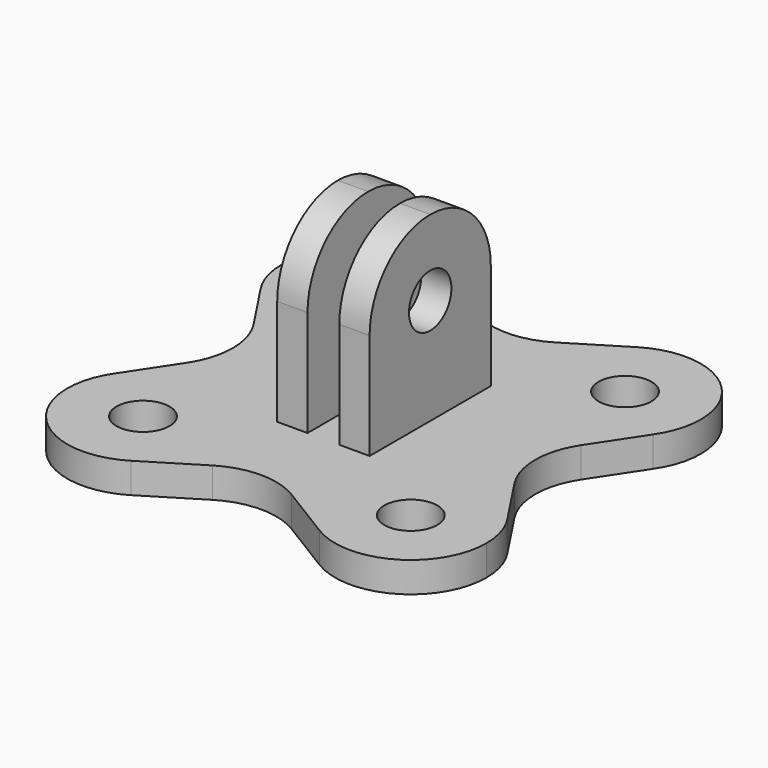
from build123d import *

# Parameters (mm, degrees)
F1_DEPTH = 12
F2_DEPTH = 2
F3_R     = 1.75
F4_DEPTH = 25
F0_R     = 1.75
F5_DEPTH = 2


# Not quite as in the source:
# - a feature names something its author has since deleted; it is built from what else it names


with BuildPart() as f1:
    # F0 (on Top) → F1 (new body)
    with BuildSketch(Plane.XY):
        Polygon((-3.05, 5), (-3.05, 0), (-3.05, -5), (-1.05, -5), (-1.05, 0), (-1.05, 5), align=None)
    extrude(amount=F1_DEPTH)


with BuildPart() as f1b:
    # F0 (on Top) → F1, piece 2 (new body)
    with BuildSketch(Plane.XY):
        Polygon((3.05, 0), (3.05, 5), (1.05, 5), (1.05, 0), (1.05, -5), (3.05, -5), align=None)
    extrude(amount=F1_DEPTH)


with BuildPart() as f2:
    # F0 (on Top) → F2 (new body)
    with BuildSketch(Plane.XY):
        Polygon((-3.05, 5), (-3.05, 0), (-3.05, -5), (-1.05, -5), (-1.05, 0), (-1.05, 5), align=None)
    extrude(amount=-F2_DEPTH)


with BuildPart() as f2b:
    # F0 (on Top) → F2, piece 2 (new body)
    with BuildSketch(Plane.XY):
        Polygon((3.05, 0), (3.05, 5), (1.05, 5), (1.05, 0), (1.05, -5), (3.05, -5), align=None)
    extrude(amount=-F2_DEPTH)


with BuildPart() as f4_tool:
    # F3 (on face) → F4 (new body)
    with BuildSketch(Plane(origin=(-3.05, 0, 0), x_dir=(0, -1, 0), z_dir=(-1, 0, 0))):
        with BuildLine():
            ThreePointArc((-5, 7), (-3.5355339059, 10.5355339059), (0, 12))
            Line((0, 12), (-5, 12))
            Line((-5, 12), (-5, 7))
        make_face()
        with Locations((0, 7)):
            Circle(F3_R)
        with BuildLine():
            ThreePointArc((0, 12), (3.5355339059, 10.5355339059), (5, 7))
            Line((5, 7), (5, 12))
            Line((5, 12), (0, 12))
        make_face()
    extrude(amount=-F4_DEPTH)


with BuildPart() as f1_1:
    add(f1.part)

    # F4: cut by f4_tool
    add(f4_tool.part, mode=Mode.SUBTRACT)


with BuildPart() as f1b_1:
    add(f1b.part)

    # F4: cut by f4_tool
    add(f4_tool.part, mode=Mode.SUBTRACT)


with BuildPart() as f5:
    # F0 (on Top) → F5 (new body)
    with BuildSketch(Plane.XY):
        with BuildLine():
            Line((10.8111245395, 2.756994834), (12.9509348337, 5.9944309568))
            ThreePointArc((12.9509348337, 5.9944309568), (12.4697533606, 12.2763382413), (6.2235598652, 13.1003294791))
            Line((6.2235598652, 13.1003294791), (2.6152748996, 10.8859287267))
            ThreePointArc((2.6152748996, 10.8859287267), (0, 10.147423441), (-2.6152748996, 10.8859287267))
            Line((-2.6152748996, 10.8859287267), (-6.2235598652, 13.1003294791))
            ThreePointArc((-6.2235598652, 13.1003294791), (-4.4755576422, 11.2805171256), (-3.8388347648, 8.8388347648))
            ThreePointArc((-3.8388347648, 8.8388347648), (-7.3489522769, 4.0659687315), (-12.9509348337, 5.9944309568))
            Line((-12.9509348337, 5.9944309568), (-10.8111245395, 2.756994834))
            ThreePointArc((-10.8111245395, 2.756994834), (-9.9823329358, 0), (-10.8111245395, -2.756994834))
            Line((-10.8111245395, -2.756994834), (-12.9509348337, -5.9944309568))
            ThreePointArc((-12.9509348337, -5.9944309568), (-7.3489522769, -4.0659687315), (-3.8388347648, -8.8388347648))
            ThreePointArc((-3.8388347648, -8.8388347648), (-4.4755576422, -11.2805171256), (-6.2235598652, -13.1003294791))
            Line((-6.2235598652, -13.1003294791), (-2.6152748996, -10.8859287267))
            ThreePointArc((-2.6152748996, -10.8859287267), (0, -10.147423441), (2.6152748996, -10.8859287267))
            Line((2.6152748996, -10.8859287267), (6.2235598652, -13.1003294791))
            ThreePointArc((6.2235598652, -13.1003294791), (5.2079161691, -5.4013312883), (12.9509348337, -5.9944309568))
            Line((12.9509348337, -5.9944309568), (10.8111245395, -2.756994834))
            ThreePointArc((10.8111245395, -2.756994834), (9.9823329358, 0), (10.8111245395, 2.756994834))
        make_face()
        Polygon((-3.05, -5), (-3.05, 0), (-3.05, 5), (-1.05, 5), (-1.05, 0), (-1.05, -5), align=None, mode=Mode.SUBTRACT)
        Polygon((1.05, 5), (3.05, 5), (3.05, 0), (3.05, -5), (1.05, -5), (1.05, 0), align=None, mode=Mode.SUBTRACT)
        with Locations((8.8388347648, 8.8388347648)):
            Circle(F0_R, mode=Mode.SUBTRACT)
        with BuildLine():
            ThreePointArc((13.8388347648, -8.8388347648), (13.6117007982, -7.3489522769), (12.9509348337, -5.9944309568))
            ThreePointArc((12.9509348337, -5.9944309568), (5.2079161691, -5.4013312883), (6.2235598652, -13.1003294791))
            ThreePointArc((6.2235598652, -13.1003294791), (11.2805171256, -13.2021118875), (13.8388347648, -8.8388347648))
        make_face()
        with Locations((8.8388347648, -8.8388347648)):
            Circle(F0_R, mode=Mode.SUBTRACT)
        with BuildLine():
            ThreePointArc((-3.8388347648, 8.8388347648), (-4.4755576422, 11.2805171256), (-6.2235598652, 13.1003294791))
            ThreePointArc((-6.2235598652, 13.1003294791), (-12.4697533606, 12.2763382413), (-12.9509348337, 5.9944309568))
            ThreePointArc((-12.9509348337, 5.9944309568), (-7.3489522769, 4.0659687315), (-3.8388347648, 8.8388347648))
        make_face()
        with Locations((-8.8388347648, 8.8388347648)):
            Circle(F0_R, mode=Mode.SUBTRACT)
        with BuildLine():
            ThreePointArc((-12.9509348337, -5.9944309568), (-12.4697533606, -12.2763382413), (-6.2235598652, -13.1003294791))
            ThreePointArc((-6.2235598652, -13.1003294791), (-4.4755576422, -11.2805171256), (-3.8388347648, -8.8388347648))
            ThreePointArc((-3.8388347648, -8.8388347648), (-7.3489522769, -4.0659687315), (-12.9509348337, -5.9944309568))
        make_face()
        with Locations((-8.8388347648, -8.8388347648)):
            Circle(F0_R, mode=Mode.SUBTRACT)
    extrude(amount=-F5_DEPTH)


solid = Compound([f2.part, f2b.part, f1_1.part, f1b_1.part, f5.part])
